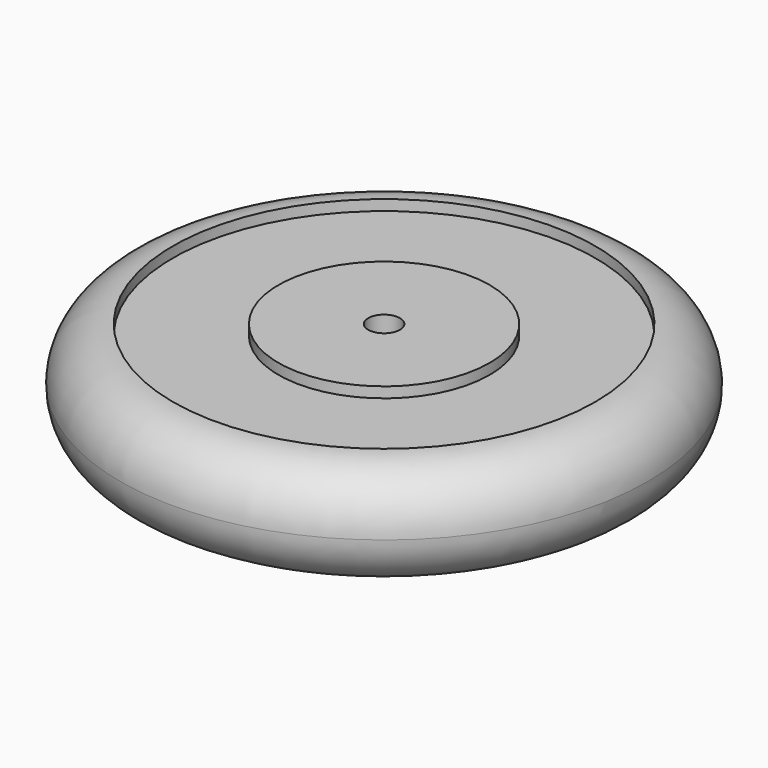
from build123d import *

# Parameters (mm, degrees)
F0_R     = 25
F0_R_2   = 20
F1_DEPTH = 5
F0_R_3   = 10
F2_DEPTH = 4
F3_R     = 4.99999
F5_D     = 3
F5_DEPTH = 250
F5_TIP   = 0.9012909285


# Not quite as in the source:
# - a fillet or chamfer is up to 0.001 mm smaller than in the source, because OpenCascade refuses the exact size


with BuildPart() as f1:
    # F0 (on Top) → F1 (new body, symmetric)
    with BuildSketch(Plane.XY):
        Circle(F0_R)
        Circle(F0_R_2, mode=Mode.SUBTRACT)
    extrude(amount=F1_DEPTH, both=True)



with BuildPart() as f1b:
    # F0 (on Top) → F1, piece 2 (new body, symmetric)
    with BuildSketch(Plane.XY):
        Circle(F0_R_3)
    extrude(amount=F1_DEPTH, both=True)


with BuildPart() as f1_1:
    add(f1.part)

    add(f1b.part)  # F2 merges F1b
    # F0 (on Top) → F2 (join, symmetric)
    with BuildSketch(Plane.XY):
        Circle(F0_R_2)
        Circle(F0_R_3, mode=Mode.SUBTRACT)
    extrude(amount=F2_DEPTH, both=True)

    # F3 (radius 5 in the source; OpenCascade refuses exactly that, so slightly less here)
    f3_edges = [f1_1.edges().sort_by_distance(p)[0] for p in [
        (-25, 0, 5),
        (-25, 0, -5),
    ]]
    fillet(f3_edges, radius=F3_R)

    # F5
    with Locations(Plane(origin=(0, 0, -5), x_dir=(1, 0, 0), z_dir=(0, 0, -1))):
        with Locations((0, 0)):
            Hole(F5_D / 2, depth=F5_DEPTH)
            with Locations((0, 0, -(F5_DEPTH + F5_TIP / 2))):  # 118° drill point
                Cone(0, F5_D / 2, F5_TIP, mode=Mode.SUBTRACT)


solid = f1_1.part
